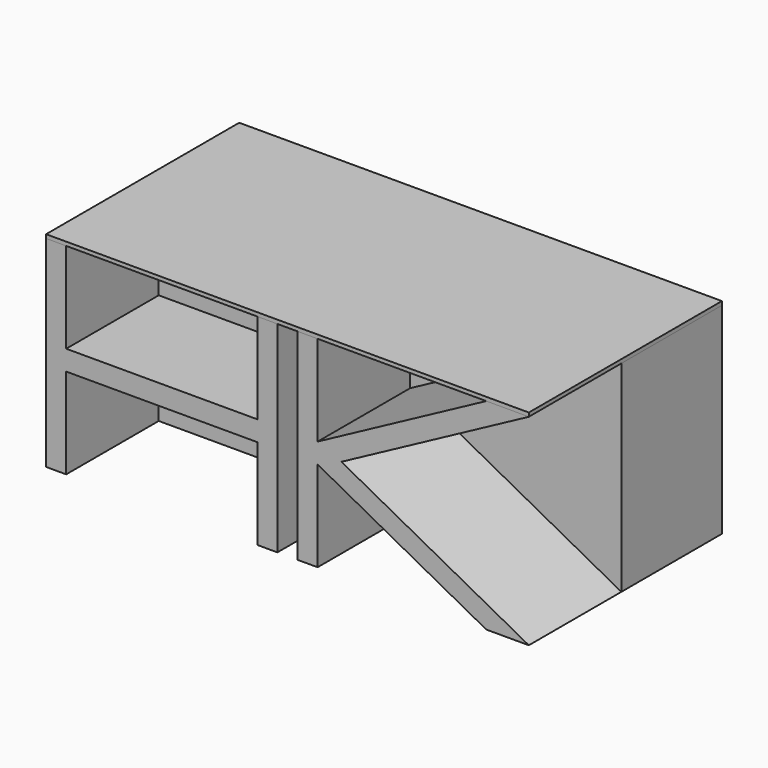
from build123d import *

# Parameters (mm, degrees)
F0_W     = 482.6
F0_H     = 228.6
F0_W_2   = 50.8
F0_H_2   = 508
F1_DEPTH = 12.7
F2_DEPTH = 304.8
F4_DEPTH = 304.8
F5_W     = 369.3403837607
F5_H     = 292.1
F5_W_2   = 50.8
F5_W_3   = 425.9701918804
F5_W_4   = 533.4
F5_W_5   = 482.6
F6_DEPTH = 9.525


# Not quite as in the source:
# - a length typed as a fraction of an inch, garbled in the dataset ("3 / 203.2 mm" for 3/8 in), is restored


with BuildPart() as f1:
    # F0 (on Front) → F1 (new body, symmetric)
    with BuildSketch(Plane.XZ):
        with Locations((-317.5, 139.7)):
            Rectangle(F0_W, F0_H)
        with Locations((-317.5, -139.7)):
            Rectangle(F0_W, F0_H)
        Polygon((-558.8, 254), (-609.6, 254), (-609.6, -254), (-558.8, -254), (-558.8, -25.4), (-76.2, -25.4), (-76.2, -254), (-25.4, -254), (-25.4, 254), (-76.2, 254), (-76.2, 25.4), (-558.8, 25.4), align=None)
        Rectangle(F0_W_2, F0_H_2)
        Polygon((76.2, 254), (25.4, 254), (25.4, -254), (76.2, -254), (76.2, -25.4), (502.1701918804, -254), (609.6, -254), (136.2997867996, 0), (609.6, 254), (502.1701918804, 254), (76.2, 25.4), align=None)
        Polygon((76.2, -25.4), (76.2, -254), (502.1701918804, -254), align=None)
        Polygon((609.6, -254), (609.6, 254), (136.2997867996, 0), align=None)
        Polygon((502.1701918804, 254), (76.2, 254), (76.2, 25.4), align=None)
    extrude(amount=F1_DEPTH, both=True)

    # F0 (on Front) → F2 (join)
    with BuildSketch(Plane.XZ):
        Polygon((-558.8, 254), (-609.6, 254), (-609.6, -254), (-558.8, -254), (-558.8, -25.4), (-76.2, -25.4), (-76.2, -254), (-25.4, -254), (-25.4, 254), (-76.2, 254), (-76.2, 25.4), (-558.8, 25.4), align=None)
        Polygon((76.2, 254), (25.4, 254), (25.4, -254), (76.2, -254), (76.2, -25.4), (502.1701918804, -254), (609.6, -254), (136.2997867996, 0), (609.6, 254), (502.1701918804, 254), (76.2, 25.4), align=None)
    extrude(amount=F2_DEPTH)

    # F3 (on Front) → F4 (join)
    with BuildSketch(Plane.XZ):
        Polygon((132.8298081196, 254), (25.4, 254), (25.4, -254), (76.2, -254), (76.2, 241.9669375636), (317.5, -38.9842283051), (558.8, 241.9669375636), (558.8, -254), (609.6, -254), (609.6, 254), (502.1701918804, 254), (317.5, 38.9842283051), align=None)
        Polygon((-25.4, -254), (-25.4, 254), (-76.2, 254), (-76.2, -203.2), (-609.6, -203.2), (-609.6, -254), align=None)
    extrude(amount=-F4_DEPTH)


with BuildPart() as f6:
    # F5 (on face) → F6 (new body)
    with BuildSketch(Plane.XY.offset(254)):
        Polygon((609.6, -12.7), (609.6, 304.8), (502.1701918804, 304.8), (502.1701918804, 12.7), (132.8298081196, 12.7), (132.8298081196, 304.8), (25.4, 304.8), (25.4, 12.7), (-25.4, 12.7), (-25.4, 304.8), (-76.2, 304.8), (-76.2, 12.7), (-609.6, 12.7), (-609.6, -304.8), (-558.8, -304.8), (-558.8, -12.7), (-76.2, -12.7), (-76.2, -304.8), (-25.4, -304.8), (-25.4, -12.7), (25.4, -12.7), (25.4, -304.8), (76.2, -304.8), (76.2, -12.7), (502.1701918804, -12.7), (502.1701918804, -304.8), (609.6, -304.8), align=None)
        with Locations((317.5, 158.75)):
            Rectangle(F5_W, F5_H)
        with Locations((0, 158.75)):
            Rectangle(F5_W_2, F5_H)
        with Locations((289.1850959402, -158.75)):
            Rectangle(F5_W_3, F5_H)
        with Locations((-342.9, 158.75)):
            Rectangle(F5_W_4, F5_H)
        with Locations((0, -158.75)):
            Rectangle(F5_W_2, F5_H)
        with Locations((-317.5, -158.75)):
            Rectangle(F5_W_5, F5_H)
    extrude(amount=F6_DEPTH)


solid = Compound([f1.part, f6.part])
